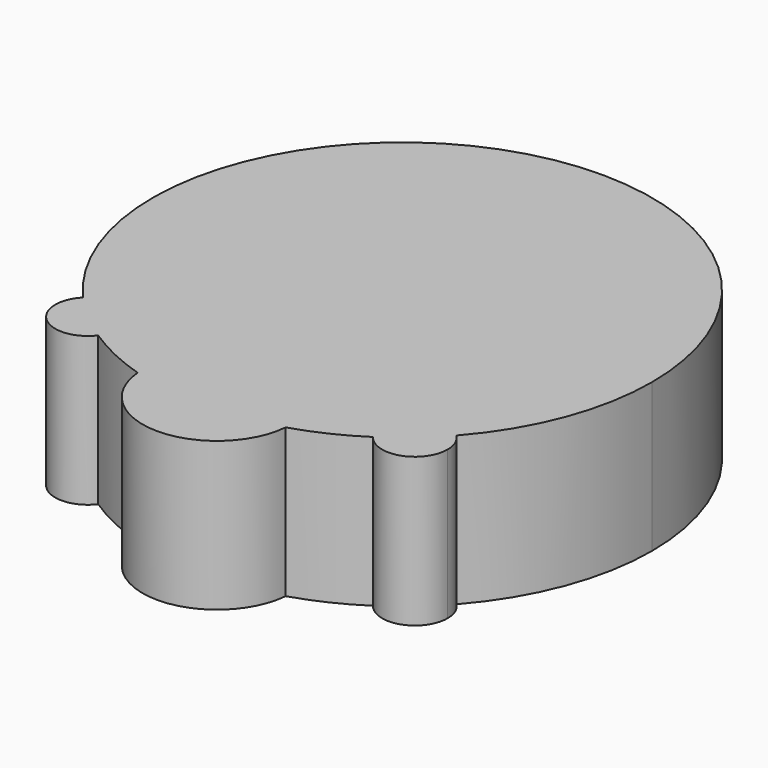
from build123d import *

# Parameters (mm, degrees)
F1_DEPTH = 25


with BuildPart() as f1:
    # F0 (on Top) → F1 (new body)
    with BuildSketch(Plane.XY):
        with BuildLine():
            ThreePointArc((31.4123807864, -27.8794249104), (39.2639783582, -14.9110698304), (42, 0))
            ThreePointArc((42, 0), (-14.9110698304, 39.2639783582), (-31.4123807864, -27.8794249104))
            ThreePointArc((-31.4123807864, -27.8794249104), (-25.4105137384, -26.6574416615), (-22, -31.7450783587))
            ThreePointArc((-22, -31.7450783587), (-22.2864690998, -33.4969617889), (-23.1160347465, -35.066350503))
            ThreePointArc((-23.1160347465, -35.066350503), (-17.9613012827, -37.9656641748), (-12.4504239602, -40.1121794872))
            ThreePointArc((-12.4504239602, -40.1121794872), (-0.5566419395, -26.5124001605), (12.5, -39))
            ThreePointArc((12.5, -39), (12.4875998395, -39.5566419395), (12.4504239602, -40.1121794872))
            ThreePointArc((12.4504239602, -40.1121794872), (17.9613012827, -37.9656641748), (23.1160347465, -35.066350503))
            ThreePointArc((23.1160347465, -35.066350503), (23.8988095238, -27.5879847641), (31.4123807864, -27.8794249104))
        make_face()
        with BuildLine():
            ThreePointArc((-22, -31.7450783587), (-25.4105137384, -26.6574416615), (-31.4123807864, -27.8794249104))
            ThreePointArc((-31.4123807864, -27.8794249104), (-27.5, -31.7450783587), (-23.1160347465, -35.066350503))
            ThreePointArc((-23.1160347465, -35.066350503), (-22.2864690998, -33.4969617889), (-22, -31.7450783587))
        make_face()
        with BuildLine():
            ThreePointArc((-23.1160347465, -35.066350503), (-27.5, -31.7450783587), (-31.4123807864, -27.8794249104))
            ThreePointArc((-31.4123807864, -27.8794249104), (-31.1011904762, -35.9021719533), (-23.1160347465, -35.066350503))
        make_face()
        with BuildLine():
            ThreePointArc((33, -31.7450783587), (32.5876366972, -29.6555920971), (31.4123807864, -27.8794249104))
            ThreePointArc((31.4123807864, -27.8794249104), (27.5, -31.7450783587), (23.1160347465, -35.066350503))
            ThreePointArc((23.1160347465, -35.066350503), (29.2518834302, -36.9586092589), (33, -31.7450783587))
        make_face()
        with BuildLine():
            ThreePointArc((23.1160347465, -35.066350503), (27.5, -31.7450783587), (31.4123807864, -27.8794249104))
            ThreePointArc((31.4123807864, -27.8794249104), (23.8988095238, -27.5879847641), (23.1160347465, -35.066350503))
        make_face()
        with BuildLine():
            ThreePointArc((12.5, -39), (-0.5566419395, -26.5124001605), (-12.4504239602, -40.1121794872))
            ThreePointArc((-12.4504239602, -40.1121794872), (0, -42), (12.4504239602, -40.1121794872))
            ThreePointArc((12.4504239602, -40.1121794872), (12.4875998395, -39.5566419395), (12.5, -39))
        make_face()
        with BuildLine():
            ThreePointArc((12.4504239602, -40.1121794872), (0, -42), (-12.4504239602, -40.1121794872))
            ThreePointArc((-12.4504239602, -40.1121794872), (0, -51.5), (12.4504239602, -40.1121794872))
        make_face()
    extrude(amount=F1_DEPTH)


solid = f1.part
